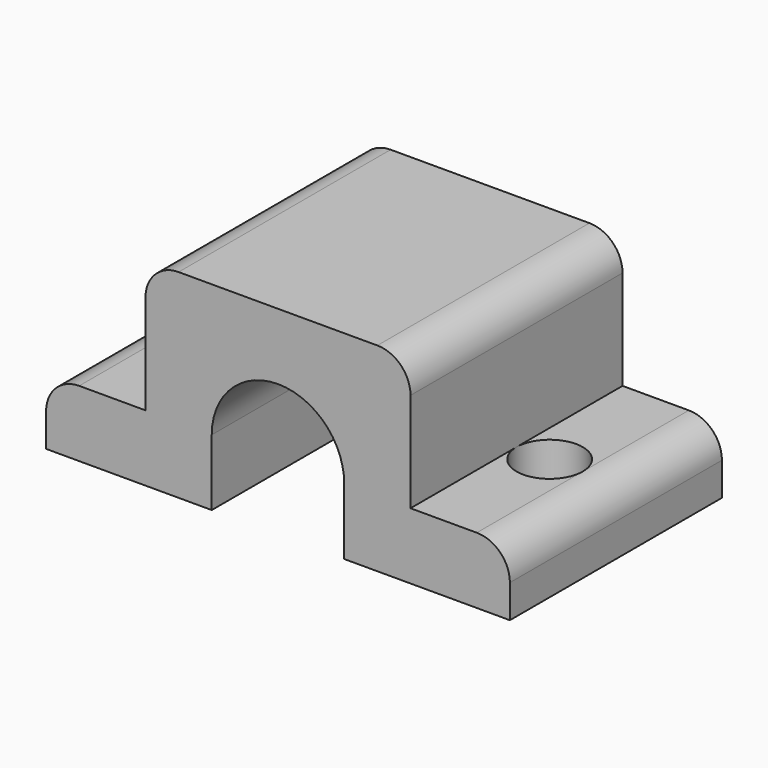
from build123d import *

# Parameters (mm, degrees)
F1_DEPTH = 8
F2_R     = 1
F3_DEPTH = 2
F4_R     = 1
F5_DEPTH = 2
F6_R     = 0.99999


# Not quite as in the source:
# - a fillet or chamfer is up to 0.001 mm smaller than in the source, because OpenCascade refuses the exact size


with BuildPart() as f1:
    # F0 (on Front) → F1 (new body)
    with BuildSketch(Plane.XZ):
        with BuildLine():
            Line((-10.1092506963, 2), (-10.1092506963, 0))
            Line((-10.1092506963, 0), (-5.1092506963, 0))
            Line((-5.1092506963, 0), (-5.1092506963, 2))
            ThreePointArc((-5.1092506963, 2), (-4.5234642587, 3.4142135624), (-3.1092506963, 4))
            ThreePointArc((-3.1092506963, 4), (-1.6950371339, 3.4142135624), (-1.1092506963, 2))
            Line((-1.1092506963, 2), (-1.1092506963, 0))
            Line((-1.1092506963, 0), (3.8907493037, 0))
            Line((3.8907493037, 0), (3.8907493037, 2))
            Line((3.8907493037, 2), (0.8907493037, 2))
            Line((0.8907493037, 2), (0.8907493037, 6))
            Line((0.8907493037, 6), (-7.1092506963, 6))
            Line((-7.1092506963, 6), (-7.1092506963, 2))
            Line((-7.1092506963, 2), (-10.1092506963, 2))
        make_face()
    extrude(amount=F1_DEPTH)

    # F2 (on face) → F3 (cut)
    with BuildSketch(Plane(origin=(0, 0, 0), x_dir=(1, 0, 0), z_dir=(0, 0, -1))):
        with Locations((-8.1092506963, 4)):
            Circle(F2_R)
    extrude(amount=-F3_DEPTH, mode=Mode.SUBTRACT)

    # F4 (on face) → F5 (cut)
    with BuildSketch(Plane(origin=(0, 0, 0), x_dir=(1, 0, 0), z_dir=(0, 0, -1))):
        with Locations((1.8907493037, 4)):
            Circle(F4_R)
    extrude(amount=-F5_DEPTH, mode=Mode.SUBTRACT)

    # F6 (radius 1 in the source; OpenCascade refuses exactly that, so slightly less here)
    f6_edges = [f1.edges().sort_by_distance(p)[0] for p in [
        (-10.109251, -4, 2),
        (-7.109251, -4, 6),
        (0.890749, -4, 6),
        (3.890749, -4, 2),
    ]]
    fillet(f6_edges, radius=F6_R)


solid = f1.part
